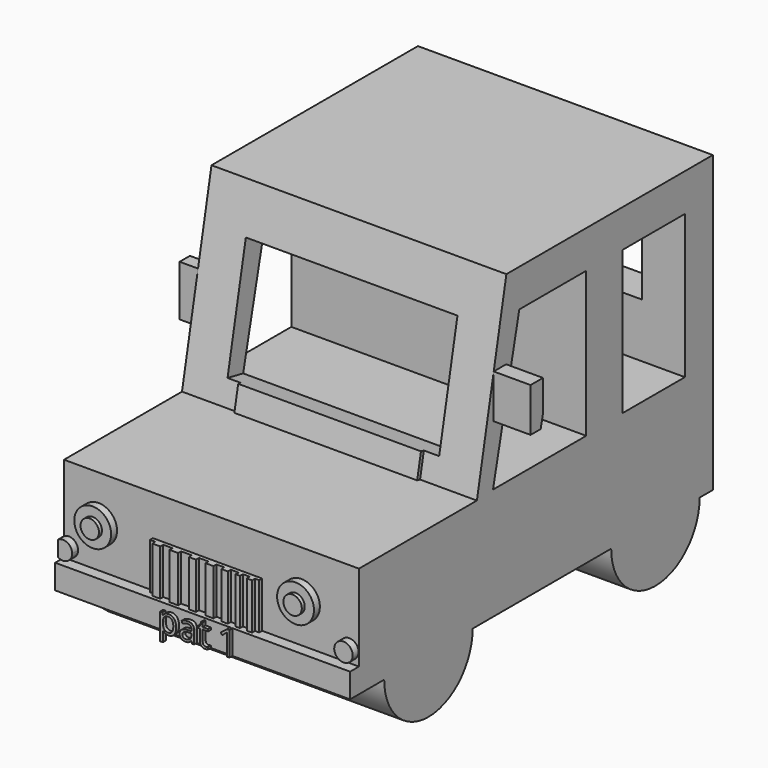
from build123d import *

# Parameters (mm, degrees)
F1_DEPTH      = 80
F2_R          = 5
F3_DEPTH      = 2
F4_W          = 57.4137987569
F4_H          = 31.6490894184
F5_DEPTH      = 25
F6_W          = 56.8318972364
F6_H          = 23.2758652419
F8_DEPTH      = 25
F7_R          = 5
F7_R_2        = 2.5
F9_DEPTH      = 2
F11_W         = 21.1422406137
F11_H         = 38.9870686922
F12_DEPTH     = 100
F13_W         = 49.593007192
F13_H         = 6.5503747573
F14_DEPTH     = 1
F15_W         = 80
F15_H         = 6.6145275188
F16_DEPTH     = 3
F17_R         = 2.5
F18_DEPTH     = 2
F19_W         = 29.6253338456
F19_H         = 12.4937789515
F20_DEPTH     = 1
F21_W         = 2.1336209029
F21_H         = 12.4937789515
F21_W_2       = 2.3275874555
F21_W_3       = 1.9396543503
F21_W_4       = 2.133615315
F21_W_5       = 1.7456896603
F21_W_6       = 1.1637955904
F21_W_7       = 1.4547407627
F22_DEPTH     = 1
F23_TEXT_SIZE = 9.1868437761
F24_DEPTH     = 1
F26_R         = 2.5
F25_R         = 2.5
F27_DEPTH     = 1
F29_DEPTH     = 5
F31_DEPTH     = 10


# Not quite as in the source:
# - Text() gives the source's letters only with a copy of the font that has no kerning and outlines rounded to 1/6400 em; it was checked with that copy


with BuildPart() as f1:
    # F0 (on Right) → F1 (new body)
    with BuildSketch(Plane.YZ):
        with BuildLine():
            ThreePointArc((25.1443261339, -27.403774525), (40.1443261339, -12.403774525), (55.1443261339, -27.403774525))
            Line((55.1443261339, -27.403774525), (59.6054219166, -27.403774525))
            Line((59.6054219166, -27.403774525), (59.6054219166, 52.596225475))
            Line((59.6054219166, 52.596225475), (-10.3945780834, 52.596225475))
            Line((-10.3945780834, 52.596225475), (-20.3945780834, 2.596225475))
            Line((-20.3945780834, 2.596225475), (-60.3945780834, 2.596225475))
            Line((-60.3945780834, 2.596225475), (-60.3945780834, -27.403774525))
            Line((-60.3945780834, -27.403774525), (-51.8258892278, -27.403774525))
            ThreePointArc((-51.8258892278, -27.403774525), (-36.8258892278, -12.403774525), (-21.8258892278, -27.403774525))
            Line((-21.8258892278, -27.403774525), (25.1443261339, -27.403774525))
        make_face()
        with BuildLine():
            ThreePointArc((-51.8258892278, -27.403774525), (-36.8258892278, -42.403774525), (-21.8258892278, -27.403774525))
            Line((-21.8258892278, -27.403774525), (-51.8258892278, -27.403774525))
        make_face()
        with BuildLine():
            Line((-51.8258892278, -27.403774525), (-21.8258892278, -27.403774525))
            ThreePointArc((-21.8258892278, -27.403774525), (-36.8258892278, -12.403774525), (-51.8258892278, -27.403774525))
        make_face()
        with BuildLine():
            ThreePointArc((25.1443261339, -27.403774525), (40.1443261339, -42.403774525), (55.1443261339, -27.403774525))
            Line((55.1443261339, -27.403774525), (25.1443261339, -27.403774525))
        make_face()
        with BuildLine():
            Line((25.1443261339, -27.403774525), (55.1443261339, -27.403774525))
            ThreePointArc((55.1443261339, -27.403774525), (40.1443261339, -12.403774525), (25.1443261339, -27.403774525))
        make_face()
    extrude(amount=F1_DEPTH)

    # F2 (on face) → F3 (join)
    with BuildSketch(Plane.XZ.offset(60.3945780834)):
        with Locations((9.37721442, -9.6833864804)):
            Circle(F2_R)
        with Locations((64.4003669485, -9.9427231839)):
            Circle(F2_R)
    extrude(amount=F3_DEPTH)

    # F4 (on face) → F5 (cut)
    with BuildSketch(Plane(origin=(0, -20.1094453638, 4.0218890728), x_dir=(1, 0, 0), z_dir=(0, -0.9805806757, 0.1961161351))):
        with Locations((40.0323285721, 20.9210221656)):
            Rectangle(F4_W, F4_H)
    extrude(amount=-F5_DEPTH, mode=Mode.SUBTRACT)

    # F6 (on face) → F8 (cut)
    with BuildSketch(Plane(origin=(0, 59.6054219166, 0), x_dir=(-1, 0, 0), z_dir=(0, 1, 0))):
        with Locations((-39.9353425018, 29.7737093642)):
            Rectangle(F6_W, F6_H)
    extrude(amount=-F8_DEPTH, mode=Mode.SUBTRACT)

    # F7 (on face) → F9 (join)
    with BuildSketch(Plane(origin=(0, 59.6054219166, 0), x_dir=(-1, 0, 0), z_dir=(0, 1, 0))):
        with Locations((-66.4884461026, -14.5383289542)):
            Circle(F7_R)
        with Locations((-55.7851432761, -15.0323286653)):
            Circle(F7_R_2)
        with Locations((-13.6305916627, -15.0323286653)):
            Circle(F7_R)
        with Locations((-25.651224153, -15.3616604882)):
            Circle(F7_R_2)
    extrude(amount=F9_DEPTH)

    # F11 (on face) → F12 (cut)
    with BuildSketch(Plane(origin=(0, 0, 0), x_dir=(0, -1, 0), z_dir=(-1, 0, 0))):
        with Locations((-39.5689662546, 22.8879310889)):
            Rectangle(F11_W, F11_H)
        Polygon((-16.6810350493, 42.4008047549), (-16.6810350493, 2.9871264132), (14.9353435263, 2.9871264132), (6.0129314661, 42.4008047549), align=None)
    extrude(amount=-F12_DEPTH, mode=Mode.SUBTRACT)

    # F13 (on face) → F14 (join)
    with BuildSketch(Plane(origin=(0, -20.1094453638, 4.0218890728), x_dir=(1, 0, 0), z_dir=(0, -0.9805806757, 0.1961161351))):
        with Locations((39.789182134, 1.8212900777)):
            Rectangle(F13_W, F13_H)
    extrude(amount=F14_DEPTH)

    # F15 (on face) → F16 (join)
    with BuildSketch(Plane.XZ.offset(60.3945780834)):
        with Locations((40, -24.0965107656)):
            Rectangle(F15_W, F15_H)
    extrude(amount=F16_DEPTH)

    # F17 (on face) → F18 (join)
    with BuildSketch(Plane.XZ.offset(60.3945780834)):
        with BuildLine():
            ThreePointArc((0, -19.9083520639), (2.5320487556, -19.9658550876), (3.8149642552, -17.7821185378))
            ThreePointArc((3.8149642552, -17.7821185378), (2.5320487556, -15.598381988), (0, -15.6558850117))
            Line((0, -15.6558850117), (0, -19.9083520639))
        make_face()
        with Locations((77.3986900343, -17.3476543278)):
            Circle(F17_R)
    extrude(amount=F18_DEPTH)

    # F19 (on face) → F20 (join)
    with BuildSketch(Plane.XZ.offset(60.3945780834)):
        with Locations((38.9212593436, -14.5423575304)):
            Rectangle(F19_W, F19_H)
    extrude(amount=F20_DEPTH)

    # F21 (on face) → F22 (join)
    with BuildSketch(Plane.XZ.offset(61.3945780834)):
        with Locations((26.6309482977, -14.5423575304)):
            Rectangle(F21_W, F21_H)
        with Locations((31.3831027597, -14.5423575304)):
            Rectangle(F21_W_2, F21_H)
        with Locations((36.4262089133, -14.5423575304)):
            Rectangle(F21_W_3, F21_H)
        with Locations((41.0813800991, -14.5423575304)):
            Rectangle(F21_W_4, F21_H)
        with Locations((45.1546553522, -14.5423575304)):
            Rectangle(F21_W_5, F21_H)
        with Locations((48.7430170178, -14.5423575304)):
            Rectangle(F21_W_6, F21_H)
        with Locations((51.8949590623, -14.5423575304)):
            Rectangle(F21_W_7, F21_H)
    extrude(amount=F22_DEPTH)

    # F23 (on face) → F24 (join)
    with BuildSketch(Plane.XZ.offset(63.3945780834)):
        with Locations((28.4938812256, -27.403774525)):
            Text('pat 1', F23_TEXT_SIZE, font='Open Sans', text_align=(TextAlign.LEFT, TextAlign.BOTTOM))
    extrude(amount=F24_DEPTH)

    # F26 (on face) + F25 (on face) → F27 (join)
    with BuildSketch(Plane.XZ.offset(62.3945780834)):
        with Locations((64.4003669485, -9.9427231839)):
            Circle(F26_R)
    with BuildSketch(Plane.XZ.offset(62.3945780834)):
        with Locations((9.37721442, -9.6833864804)):
            Circle(F25_R)
    extrude(amount=F27_DEPTH)

    # F28 (on face) → F29 (join)
    with BuildSketch(Plane(origin=(0, 0, 0), x_dir=(0, -1, 0), z_dir=(-1, 0, 0))):
        Polygon((14.9539317936, 29.7737084329), (11.4625534043, 29.7737084329), (11.4625534043, 18.3277576118), (11.9890198029, 16.0021558404), (14.9539317936, 16.0021558404), align=None)
    extrude(amount=F29_DEPTH)

    # F30 (on face) → F31 (join)
    with BuildSketch(Plane.YZ.offset(80)):
        Polygon((-10.4741374962, 31.1086150686), (-14.6921001647, 31.1086150686), (-14.6921001647, 19.2049778998), (-11.2639695317, 19.2049778998), (-10.4741374962, 22.693965584), align=None)
    extrude(amount=F31_DEPTH)


solid = f1.part
